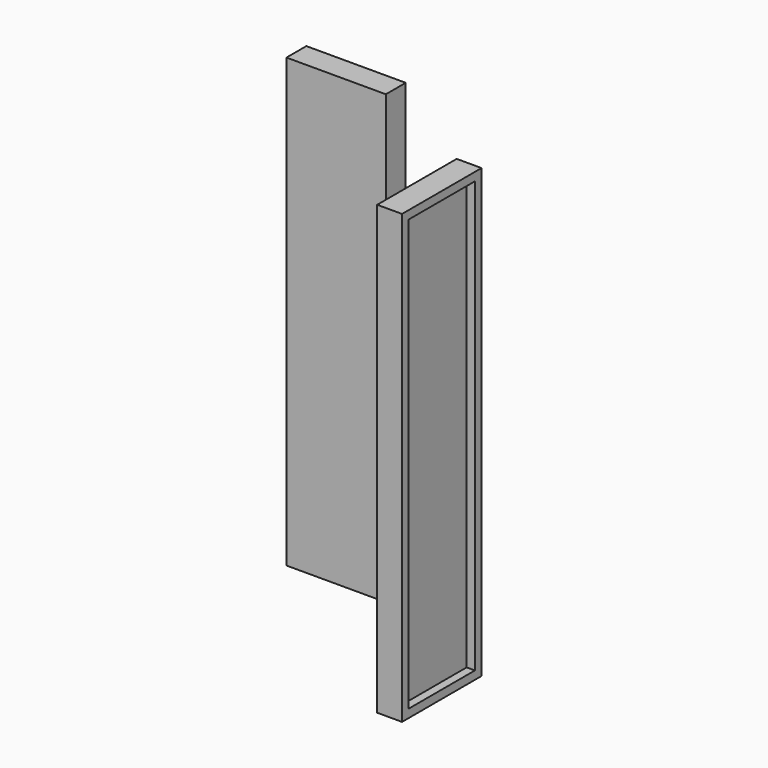
from build123d import *

# Parameters (mm, degrees)
F0_W     = 60
F0_H     = 270
F2_DEPTH = 15
F3_W     = 50
F3_H     = 260
F4_DEPTH = 5
F1_W     = 60
F1_H     = 270
F5_DEPTH = 15
F6_W     = 50
F6_H     = 260
F7_DEPTH = 5
F9_DEPTH = 10


# Not quite as in the source:
# - a feature names something its author has since deleted; it is built from what else it names


with BuildPart() as f2:
    # F0 (on Front) → F2 (new body)
    with BuildSketch(Plane.XZ):
        with Locations((-121.8493213905, -25.8904273567)):
            Rectangle(F0_W, F0_H)
    extrude(amount=F2_DEPTH)

    # F3 (on face) → F4 (join)
    with BuildSketch(Plane.XZ):
        with Locations((-121.8493213905, -25.8904273567)):
            Rectangle(F3_W, F3_H)
    extrude(amount=-F4_DEPTH)

    # F8 (on face) → F9 (cut)
    with BuildSketch(Plane(origin=(0, 5, 0), x_dir=(-1, 0, 0), z_dir=(0, 1, 0))):
        with BuildLine():
            Line((109.8493213905, -150.8904273567), (133.8493213905, -150.8904273567))
            Line((133.8493213905, -150.8904273567), (133.8493213905, -45.8904273567))
            add(Edge.make_bspline(
                [(109.8493213905, -45.8904273567), (121.8493213905, -57.1404273567), (133.8493213905, -45.8904273567)],
                knots=[2.4980915448, 2.4980915448, 2.4980915448, 3.7850937624, 3.7850937624, 3.7850937624], degree=2, weights=[1, 0.8, 1]))
            Line((109.8493213905, -45.8904273567), (109.8493213905, -150.8904273567))
        make_face()
        with BuildLine():
            add(Edge.make_bspline(
                [(133.8493213905, -5.8904273567), (128.5159880572, -0.8904273567), (121.8493213905, -0.8904273567)],
                knots=[5.6396841984, 5.6396841984, 5.6396841984, 6.2831853072, 6.2831853072, 6.2831853072], degree=2, weights=[1, 0.9486832981, 1]))
            Line((133.8493213905, -5.8904273567), (133.8493213905, 99.1095726433))
            Line((133.8493213905, 99.1095726433), (109.8493213905, 99.1095726433))
            Line((109.8493213905, 99.1095726433), (109.8493213905, -5.8904273567))
            add(Edge.make_bspline(
                [(121.8493213905, -0.8904273567), (115.1826547239, -0.8904273567), (109.8493213905, -5.8904273567)],
                knots=[0, 0, 0, 0.6435011088, 0.6435011088, 0.6435011088], degree=2, weights=[1, 0.9486832981, 1]))
        make_face()
        with BuildLine():
            Line((133.8493213905, -5.8904273567), (133.8493213905, -45.8904273567))
            add(Edge.make_bspline(
                [(133.8493213905, -45.8904273567), (155.1826547239, -25.8904273567), (133.8493213905, -5.8904273567)],
                knots=[3.7850937624, 3.7850937624, 3.7850937624, 5.6396841984, 5.6396841984, 5.6396841984], degree=2, weights=[1, 0.6, 1]))
        make_face()
        with BuildLine():
            add(Edge.make_bspline(
                [(109.8493213905, -45.8904273567), (121.8493213905, -57.1404273567), (133.8493213905, -45.8904273567)],
                knots=[2.4980915448, 2.4980915448, 2.4980915448, 3.7850937624, 3.7850937624, 3.7850937624], degree=2, weights=[1, 0.8, 1]))
            Line((133.8493213905, -45.8904273567), (133.8493213905, -5.8904273567))
            add(Edge.make_bspline(
                [(133.8493213905, -5.8904273567), (128.5159880572, -0.8904273567), (121.8493213905, -0.8904273567)],
                knots=[5.6396841984, 5.6396841984, 5.6396841984, 6.2831853072, 6.2831853072, 6.2831853072], degree=2, weights=[1, 0.9486832981, 1]))
            add(Edge.make_bspline(
                [(121.8493213905, -0.8904273567), (115.1826547239, -0.8904273567), (109.8493213905, -5.8904273567)],
                knots=[0, 0, 0, 0.6435011088, 0.6435011088, 0.6435011088], degree=2, weights=[1, 0.9486832981, 1]))
            Line((109.8493213905, -5.8904273567), (109.8493213905, -45.8904273567))
        make_face()
        with BuildLine():
            add(Edge.make_bspline(
                [(109.8493213905, -5.8904273567), (88.5159880572, -25.8904273567), (109.8493213905, -45.8904273567)],
                knots=[0.6435011088, 0.6435011088, 0.6435011088, 2.4980915448, 2.4980915448, 2.4980915448], degree=2, weights=[1, 0.6, 1]))
            Line((109.8493213905, -45.8904273567), (109.8493213905, -5.8904273567))
        make_face()
    extrude(amount=-F9_DEPTH, mode=Mode.SUBTRACT)


with BuildPart() as f5:
    # F1 (on Right) → F5 (new body)
    with BuildSketch(Plane.YZ):
        with Locations((-106.3447256267, -5.4207965732)):
            Rectangle(F1_W, F1_H)
    extrude(amount=F5_DEPTH)

    # F6 (on face) → F7 (cut)
    with BuildSketch(Plane.YZ.offset(15)):
        with Locations((-106.3447256267, -5.4207965732)):
            Rectangle(F6_W, F6_H)
    extrude(amount=-F7_DEPTH, mode=Mode.SUBTRACT)


solid = Compound([f2.part, f5.part])
